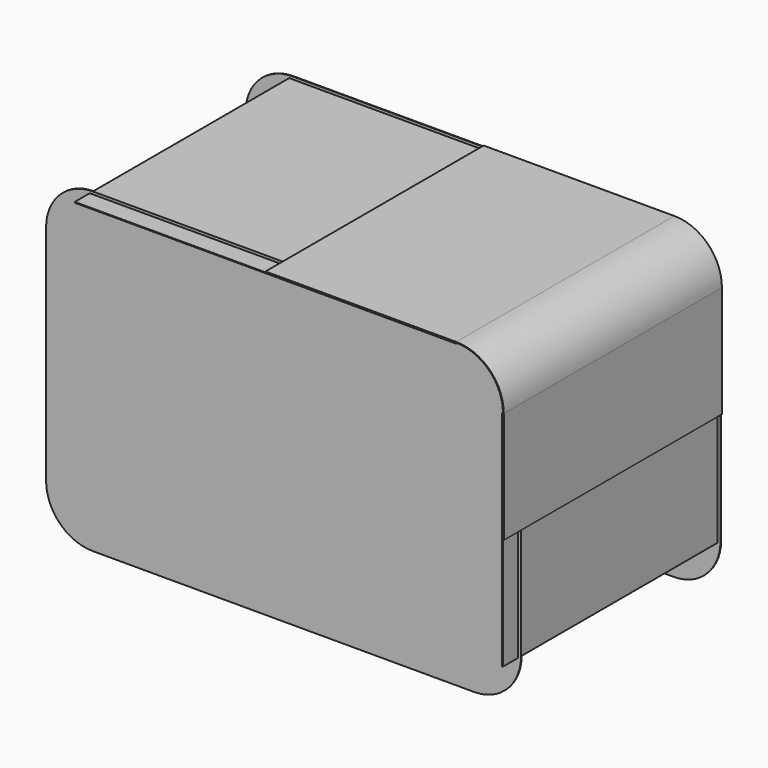
from build123d import *

# Parameters (mm, degrees)
F2_DEPTH = 350
F1_W     = 244.8
F1_H     = 1
F3_DEPTH = 314
F1_W_2   = 1
F1_H_2   = 143.2
F5_DEPTH = 24
F7_DEPTH = 1


# Not quite as in the source:
# - a feature names something its author has since deleted; it is built from what else it names


with BuildPart() as f2:
    # F1 (on Front) → F2 (new body)
    with BuildSketch(Plane.XZ):
        with BuildLine():
            Line((0, 203.2), (244.8, 203.2))
            ThreePointArc((244.8, 203.2), (287.2264068712, 185.6264068712), (304.8, 143.2))
            Line((304.8, 143.2), (304.8, 0))
            Line((304.8, 0), (305.8, 0))
            Line((305.8, 0), (305.8, 143.2))
            ThreePointArc((305.8, 143.2), (287.9335136524, 186.3335136524), (244.8, 204.2))
            Line((244.8, 204.2), (0, 204.2))
            Line((0, 204.2), (0, 203.2))
        make_face()
    extrude(amount=F2_DEPTH)


with BuildPart() as f3:
    # F1 (on Front) → F3 (new body)
    with BuildSketch(Plane.XZ):
        with Locations((122.4, 202.7)):
            Rectangle(F1_W, F1_H)
        with Locations((-122.4, 202.7)):
            Rectangle(F1_W, F1_H)
    extrude(amount=F3_DEPTH)


with BuildPart() as f3b:
    # F1 (on Front) → F3, piece 2 (new body)
    with BuildSketch(Plane.XZ):
        with Locations((304.3, 71.6)):
            Rectangle(F1_W_2, F1_H_2)
        with Locations((304.3, -71.6)):
            Rectangle(F1_W_2, F1_H_2)
    extrude(amount=F3_DEPTH)


with BuildPart() as f3_1:
    # F4: moved
    add(f3.part.moved(Location((0, -6, 0))))


with BuildPart() as f3b_1:
    # F4: moved
    add(f3b.part.moved(Location((0, -6, 0))))


with BuildPart() as f5:
    # F1 (on Front) → F5 (new body)
    with BuildSketch(Plane.XZ):
        with Locations((122.4, 202.7)):
            Rectangle(F1_W, F1_H)
        with Locations((-122.4, 202.7)):
            Rectangle(F1_W, F1_H)
    extrude(amount=F5_DEPTH)


with BuildPart() as f5b:
    # F1 (on Front) → F5, piece 2 (new body)
    with BuildSketch(Plane.XZ):
        with Locations((304.3, 71.6)):
            Rectangle(F1_W_2, F1_H_2)
        with Locations((304.3, -71.6)):
            Rectangle(F1_W_2, F1_H_2)
    extrude(amount=F5_DEPTH)


with BuildPart() as f5b_1:
    # F6: moved
    add(f5b.part.moved(Location((0, -326, 0))))


with BuildPart() as f5_1:
    # F6: moved
    add(f5.part.moved(Location((0, -326, 0))))


with BuildPart() as f7:
    # F1 (on Front) → F7 (new body)
    with BuildSketch(Plane.XZ):
        with Locations((122.4, 202.7)):
            Rectangle(F1_W, F1_H)
        with BuildLine():
            ThreePointArc((304.8, 143.2), (287.2264068712, 185.6264068712), (244.8, 203.2))
            Line((244.8, 203.2), (244.8, 202.2))
            Line((244.8, 202.2), (0, 202.2))
            Line((0, 202.2), (0, 0))
            Line((0, 0), (303.8, 0))
            Line((303.8, 0), (303.8, 143.2))
            Line((303.8, 143.2), (304.8, 143.2))
        make_face()
        with Locations((304.3, 71.6)):
            Rectangle(F1_W_2, F1_H_2)
        with Locations((-122.4, 202.7)):
            Rectangle(F1_W, F1_H)
        Polygon((-303.8, 143.2), (-304.8, 143.2), (-304.8, 0), (-304.8, -143.2), (-303.8, -143.2), (-303.8, 0), align=None)
        Polygon((0, -203.2), (244.8, -203.2), (244.8, -202.2), (0, -202.2), (-244.8, -202.2), (-244.8, -203.2), align=None)
        with Locations((304.3, -71.6)):
            Rectangle(F1_W_2, F1_H_2)
        with BuildLine():
            Line((0, 0), (0, 202.2))
            Line((0, 202.2), (-244.8, 202.2))
            Line((-244.8, 202.2), (-244.8, 203.2))
            ThreePointArc((-244.8, 203.2), (-287.2264068712, 185.6264068712), (-304.8, 143.2))
            Line((-304.8, 143.2), (-303.8, 143.2))
            Line((-303.8, 143.2), (-303.8, 0))
            Line((-303.8, 0), (-303.8, -143.2))
            Line((-303.8, -143.2), (-304.8, -143.2))
            ThreePointArc((-304.8, -143.2), (-287.2264068712, -185.6264068712), (-244.8, -203.2))
            Line((-244.8, -203.2), (-244.8, -202.2))
            Line((-244.8, -202.2), (0, -202.2))
            Line((0, -202.2), (244.8, -202.2))
            Line((244.8, -202.2), (244.8, -203.2))
            ThreePointArc((244.8, -203.2), (287.2264068712, -185.6264068712), (304.8, -143.2))
            Line((304.8, -143.2), (303.8, -143.2))
            Line((303.8, -143.2), (303.8, 0))
            Line((303.8, 0), (0, 0))
        make_face()
    extrude(amount=F7_DEPTH)


with BuildPart() as f8_1:
    # F8: copy of F7
    add(f7.part.moved(Location((0, -320, 0))))


solid = Compound([f2.part, f3_1.part, f3b_1.part, f5b_1.part, f5_1.part, f7.part, f8_1.part])
